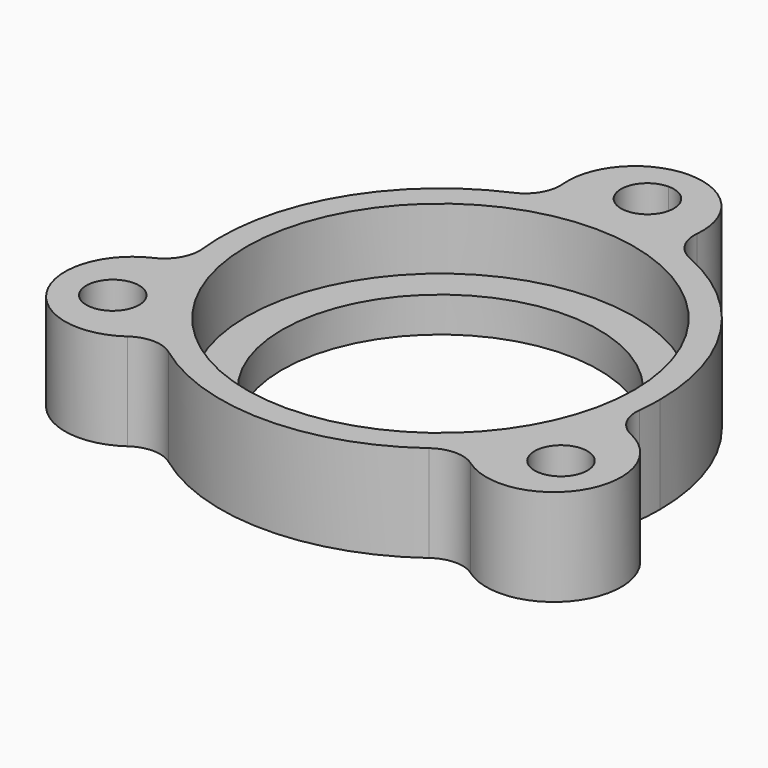
from build123d import *

# Parameters (mm, degrees)
F0_R     = 1.5
F0_R_2   = 11.025
F1_DEPTH = 5.5
F0_R_3   = 9
F2_DEPTH = 2
F3_R     = 2


with BuildPart() as f1:
    # F0 (on Top) → F1 (new body)
    with BuildSketch(Plane.XY):
        with BuildLine():
            ThreePointArc((-12.1141484076, -3.0817865531), (-15.3023705753, -8.8348277709), (-8.7259796478, -8.9502669896))
            ThreePointArc((-8.7259796478, -8.9502669896), (-10.8253175473, -6.25), (-12.1141484076, -3.0817865531))
        make_face()
        with Locations((-12.7438917843, -7.3576893522)):
            Circle(F0_R, mode=Mode.SUBTRACT)
        with BuildLine():
            ThreePointArc((12.1141484076, -3.0817865531), (12.403161998, -1.5529238399), (12.5, 0))
            ThreePointArc((12.5, 0), (9.9649914575, 7.5464524945), (3.3881687598, 12.0320535427))
            ThreePointArc((3.3881687598, 12.0320535427), (1.7101653013, 12.3824607668), (0, 12.5))
            ThreePointArc((0, 12.5), (-1.7101653013, 12.3824607668), (-3.3881687598, 12.0320535427))
            ThreePointArc((-3.3881687598, 12.0320535427), (-10.8253175473, 6.25), (-12.1141484076, -3.0817865531))
            ThreePointArc((-12.1141484076, -3.0817865531), (-10.8253175473, -6.25), (-8.7259796478, -8.9502669896))
            ThreePointArc((-8.7259796478, -8.9502669896), (0, -12.5), (8.7259796478, -8.9502669896))
            ThreePointArc((8.7259796478, -8.9502669896), (10.8253175473, -6.25), (12.1141484076, -3.0817865531))
        make_face()
        Circle(F0_R_2, mode=Mode.SUBTRACT)
        with BuildLine():
            ThreePointArc((-3.3881687598, 12.0320535427), (-1.7101653013, 12.3824607668), (0, 12.5))
            Line((0, 12.5), (0, 13.2153787043))
            ThreePointArc((0, 13.2153787043), (-1.5, 14.7153787043), (0, 16.2153787043))
            Line((0, 16.2153787043), (0, 16.9307574087))
            Line((0, 16.9307574087), (0, 17.6696555418))
            ThreePointArc((0, 17.6696555418), (-3.2887020177, 15.8092112452), (-3.3881687598, 12.0320535427))
        make_face()
        with BuildLine():
            ThreePointArc((0, 12.5), (1.7101653013, 12.3824607668), (3.3881687598, 12.0320535427))
            ThreePointArc((3.3881687598, 12.0320535427), (3.2887020177, 15.8092112452), (0, 17.6696555418))
            Line((0, 17.6696555418), (0, 16.9307574087))
            Line((0, 16.9307574087), (0, 16.2153787043))
            ThreePointArc((0, 16.2153787043), (1.0606601718, 15.7760388761), (1.5, 14.7153787043))
            ThreePointArc((1.5, 14.7153787043), (1.0606601718, 13.6547185326), (0, 13.2153787043))
            Line((0, 13.2153787043), (0, 12.5))
        make_face()
        with BuildLine():
            ThreePointArc((8.7259796478, -8.9502669896), (15.3023705753, -8.8348277709), (12.1141484076, -3.0817865531))
            ThreePointArc((12.1141484076, -3.0817865531), (10.8253175473, -6.25), (8.7259796478, -8.9502669896))
        make_face()
        with Locations((12.7438917843, -7.3576893522)):
            Circle(F0_R, mode=Mode.SUBTRACT)
    extrude(amount=F1_DEPTH)

    # F0 (on Top) → F2 (join)
    with BuildSketch(Plane.XY):
        Circle(F0_R_2)
        Circle(F0_R_3, mode=Mode.SUBTRACT)
    extrude(amount=F2_DEPTH)

    # F3
    f3_edges = [f1.edges().sort_by_distance(p)[0] for p in [
        (3.388169, 12.032054, 2.75),
        (8.72598, -8.950267, 2.75),
        (-12.114148, -3.081787, 2.75),
        (-8.72598, -8.950267, 2.75),
        (-3.388169, 12.032054, 2.75),
        (12.114148, -3.081787, 2.75),
    ]]
    fillet(f3_edges, radius=F3_R)


solid = f1.part
